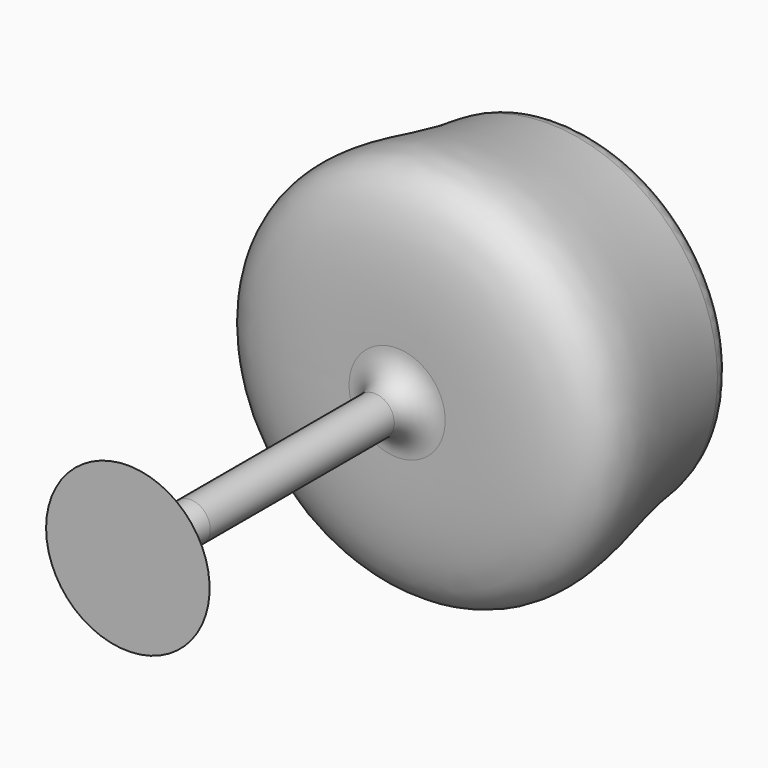
from build123d import *

# Parameters (mm, degrees)
F2_R = 5.08
F3_T = 2.54


# Not quite as in the source:
# - a shell that OpenCascade refuses in one call is made with other operations: the cavity is built on its own and cut out


with BuildPart() as f1:
    # F0 (on Top) → F1 (revolve)
    with BuildSketch(Plane.XY):
        with BuildLine():
            Line((-4.4621749899, -6.4548418265), (-4.4621749899, -58.5150425204))
            ThreePointArc((-4.4621749899, -58.5150425204), (-4.3360837237, -61.0427959336), (-3.9590618153, -63.5454526832))
            add(Edge.make_bspline(
                [(-3.9590618153, -63.5454526832), (-3.4482239959, -66.073729894), (-2.9289890524, -72.5070184577), (-12.4943527332, -74.7956886465), (-18.4944327921, -76.2313062371)],
                knots=[0.0983943665, 0.0983943665, 0.0983943665, 0.0983943665, 0.4344484786, 1, 1, 1, 1], degree=3))
            Line((-18.4944327921, -76.2313062371), (0, -76.2313062371))
            Line((0, -76.2313062371), (0, 47.1574812874))
            Line((0, 47.1574812874), (-38.1, 47.1574812874))
            add(Edge.make_bspline(
                [(-10.8753399986, -0.1051559932), (-24.0804030891, -0.2365164961), (-53.8867917052, 1.1972984925), (-38.1790002619, 30.9945182712), (-38.1, 47.1574812874)],
                knots=[0.0692152754, 0.0692152754, 0.0692152754, 0.0692152754, 0.4921599265, 1, 1, 1, 1], degree=3))
            ThreePointArc((-10.8753399986, -0.1051559932), (-6.3444349463, -1.9424368245), (-4.4621749899, -6.4548418265))
        make_face()
    revolve(axis=Axis((0, -14.5369124748, 0), (0, -1, 0)))

    # F2
    f2_edges = [f1.edges().sort_by_distance(p)[0] for p in [
        (38.1, 47.157481, 0),
        (10.87534, -0.105156, 0),
        (-43.141323, 10.778526, 0),
    ]]
    fillet(f2_edges, radius=F2_R)

    # F3: shell of thickness 2.54, made by hand


with BuildPart() as f3_core1:
    # F3_t2: copy of F1
    add(f1.part)

    # the walls: a layer under each face that stays
    f3_faces = [f3_core1.faces().sort_by_distance(p)[0] for p in [
        (36.6980535185, 45.8320109386, 0),
        (42.2566325914, 7.7991455605, 0),
        (6.3444349463, -1.9424368245, 0),
        (4.4621749899, -32.4849421735, 0),
        (4.3360837237, -61.0427959336, 0),
        (6.1560032358, -71.9723790145, 0),
        (0, -76.2313062371, 0),
    ]]
    thicken(f3_faces, amount=-F3_T, mode=Mode.SUBTRACT)


with BuildPart() as f1_1:
    add(f1.part)

    # what is left inside the walls is the cavity
    f3_cavity = [f3_core1.part.solids().sort_by_distance(p)[0] for p in [
        (34.731064, 4.861232, 0),
    ]]
    add(f3_cavity, mode=Mode.SUBTRACT)


solid = f1_1.part
